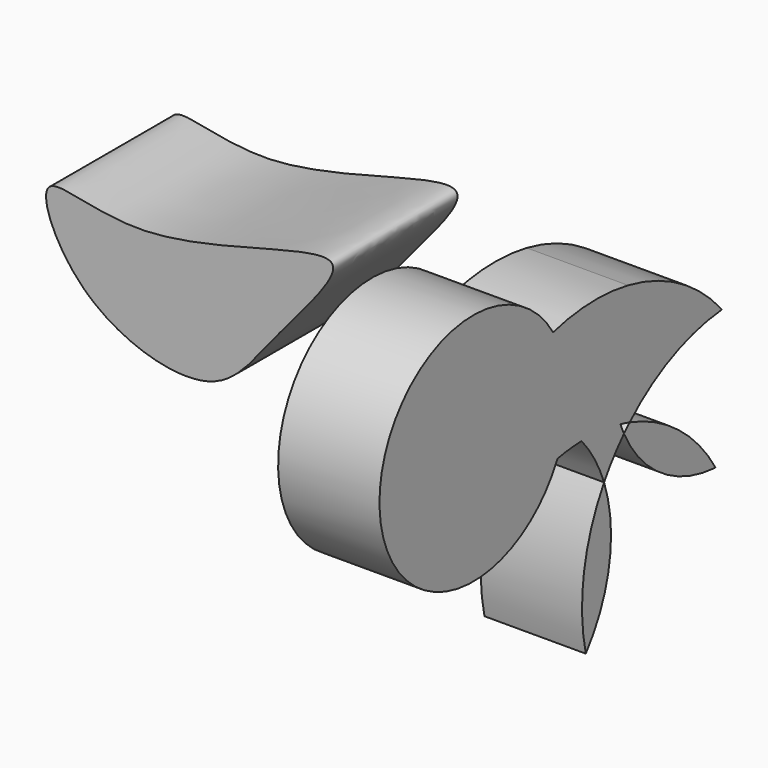
from build123d import *

# Parameters (mm, degrees)
F1_DEPTH = 16.3
F3_DEPTH = 25


with BuildPart() as f1:
    # F0 (on Right) → F1 (new body)
    with BuildSketch(Plane.YZ):
        with BuildLine():
            ThreePointArc((-12.1971222107, 45.0054410083), (-11.7748566709, 47.2766931346), (-11.6333942401, 49.5825298131))
            ThreePointArc((-11.6333942401, 49.5825298131), (-12.3508619293, 54.7354751662), (-14.44868705, 59.4964346767))
            ThreePointArc((-14.44868705, 59.4964346767), (-23.1935215297, 55.7063236123), (-30.496686697, 49.5825298131))
            ThreePointArc((-30.496686697, 49.5825298131), (-20.8754452172, 49.1789168751), (-12.1971222107, 45.0054410083))
        make_face()
        with BuildLine():
            ThreePointArc((-14.44868705, 59.4964346767), (-12.3508619293, 54.7354751662), (-11.6333942401, 49.5825298131))
            ThreePointArc((-11.6333942401, 49.5825298131), (-11.7748566709, 47.2766931346), (-12.1971222107, 45.0054410083))
            ThreePointArc((-12.1971222107, 45.0054410083), (-10.3881149892, 43.4784974996), (-8.7393013606, 41.7798282486))
            ThreePointArc((-8.7393013606, 41.7798282486), (-4.8040885537, 41.6369515569), (-0.9201595956, 40.987790996))
            ThreePointArc((-0.9201595956, 40.987790996), (-2.3378643948, 50.6817460292), (0.6132117717, 60.0237908024))
            ThreePointArc((0.6132117717, 60.0237908024), (-6.9481373655, 60.6283639636), (-14.44868705, 59.4964346767))
        make_face()
        with BuildLine():
            ThreePointArc((-30.496686697, 49.5825298131), (-23.1935215297, 55.7063236123), (-14.44868705, 59.4964346767))
            ThreePointArc((-14.44868705, 59.4964346767), (-46.7573242092, 59.1436735736), (-31.357916302, 30.7389079244))
            ThreePointArc((-31.357916302, 30.7389079244), (-23.3830823555, 37.5506109415), (-13.5710991485, 41.2549678377))
            ThreePointArc((-13.5710991485, 41.2549678377), (-12.7845624252, 43.0937351564), (-12.1971222107, 45.0054410083))
            ThreePointArc((-12.1971222107, 45.0054410083), (-20.8754452172, 49.1789168751), (-30.496686697, 49.5825298131))
        make_face()
        with BuildLine():
            ThreePointArc((-8.7393013606, 41.7798282486), (-10.3881149892, 43.4784974996), (-12.1971222107, 45.0054410083))
            ThreePointArc((-12.1971222107, 45.0054410083), (-12.7845624252, 43.0937351564), (-13.5710991485, 41.2549678377))
            ThreePointArc((-13.5710991485, 41.2549678377), (-11.1656812919, 41.6138851313), (-8.7393013606, 41.7798282486))
        make_face()
        with BuildLine():
            ThreePointArc((-13.5710991485, 41.2549678377), (-23.3830823555, 37.5506109415), (-31.357916302, 30.7389079244))
            ThreePointArc((-31.357916302, 30.7389079244), (-20.8965420075, 33.3448876118), (-13.5710991485, 41.2549678377))
        make_face()
        with BuildLine():
            ThreePointArc((19.4906238467, 48.9234365523), (10.9960641192, 56.0792416197), (0.6132117717, 60.0237908024))
            ThreePointArc((0.6132117717, 60.0237908024), (-2.3378643948, 50.6817460292), (-0.9201595956, 40.987790996))
            ThreePointArc((-0.9201595956, 40.987790996), (0.0090353267, 40.7544944765), (0.9304370528, 40.4921029198))
            ThreePointArc((0.9304370528, 40.4921029198), (9.4956537387, 46.2814526039), (19.4906238467, 48.9234365523))
        make_face()
        with BuildLine():
            ThreePointArc((-0.9201595956, 40.987790996), (-4.8040885537, 41.6369515569), (-8.7393013606, 41.7798282486))
            ThreePointArc((-8.7393013606, 41.7798282486), (-6.1075185605, 38.1452977309), (-4.2026985521, 34.0823242475))
            ThreePointArc((-4.2026985521, 34.0823242475), (-2.3451015259, 36.82323), (-0.2050463277, 39.3497681066))
            ThreePointArc((-0.2050463277, 39.3497681066), (-0.5793209757, 40.1614809514), (-0.9201595956, 40.987790996))
        make_face()
    extrude(amount=F1_DEPTH)


with BuildPart() as f1b:
    # F0 (on Right) → F1, piece 2 (new body)
    with BuildSketch(Plane.YZ):
        with BuildLine():
            ThreePointArc((-7.8750019893, 11.3203125075), (-3.1073807878, 22.228370486), (-4.2026985521, 34.0823242475))
            ThreePointArc((-4.2026985521, 34.0823242475), (-8.2400086329, 23.0564417081), (-7.8750019893, 11.3203125075))
        make_face()
    extrude(amount=F1_DEPTH)


with BuildPart() as f1c:
    # F0 (on Right) → F1, piece 3 (new body)
    with BuildSketch(Plane.YZ):
        with BuildLine():
            ThreePointArc((-0.2050463277, 39.3497681066), (7.3379322182, 30.7056804526), (18.216154673, 27.0613625553))
            ThreePointArc((18.216154673, 27.0613625553), (10.8209680209, 35.382519762), (0.9304370528, 40.4921029198))
            ThreePointArc((0.9304370528, 40.4921029198), (0.3552553346, 39.9283309178), (-0.2050463277, 39.3497681066))
        make_face()
    extrude(amount=F1_DEPTH)


with BuildPart() as f3:
    # F2 (on Front) → F3 (new body)
    with BuildSketch(Plane.XZ):
        with BuildLine():
            add(Edge.make_bspline(
                [(-50.7769659162, 48.1923893094), (-55.2717001004, 52.5799209169), (-60.455203499, 65.4338519193), (-41.1479753801, 54.8614513769), (-1.0840439012, 71.9976398536), (-21.2575691949, 50.6511793978), (-29.2422220069, 37.8950901924), (-45.221630707, 42.7695527586), (-50.7769659162, 48.1923893094)],
                knots=[0, 0, 0, 0, 0.1441466285, 0.2977703205, 0.5138029535, 0.66851698, 0.8218397779, 1, 1, 1, 1], degree=3))
        make_face()
    extrude(amount=F3_DEPTH)


solid = Compound([f1.part, f1b.part, f1c.part, f3.part])
